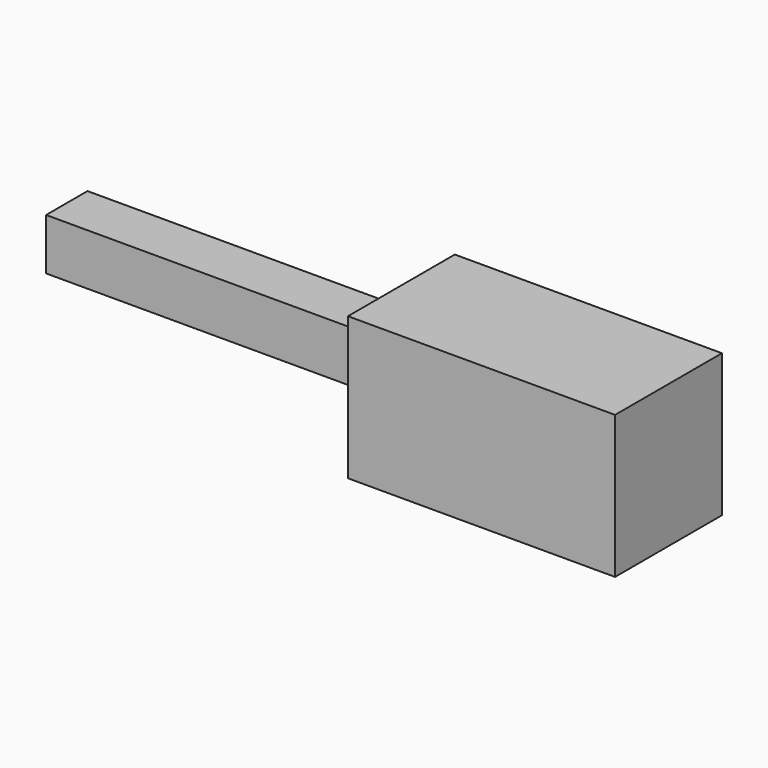
from build123d import *

# Parameters (mm, degrees)
F0_W     = 50.8
F0_H     = 27.1318203053
F1_DEPTH = 25.4
F2_DEPTH = 25.4
F4_W     = 9.8461210728
F4_H     = 9.7858998924
F5_DEPTH = 62.9539089


# Not quite as in the source:
# - an extrude ends at something that could not be found from the text; its depth is read off the source's solid


with BuildPart() as f1:
    # F0 (on Front) → F1 (new body)
    with BuildSketch(Plane.XZ):
        with Locations((-45.1160669327, 19.4199038669)):
            Rectangle(F0_W, F0_H)
    extrude(amount=F1_DEPTH)

    # F2 (add): a face of the model
    f2_faces = [f1.faces().sort_by_distance(p)[0] for p in [
        (-70.5160669327, -12.7, 19.4199038669),
    ]]
    extrude(f2_faces, amount=-F2_DEPTH)

    # F4 (on face) → F5 (join, through all)
    with BuildSketch(Plane(origin=(-70.5160669327, 0, 0), x_dir=(0, -1, 0), z_dir=(-1, 0, 0))):
        with Locations((13.5363917798, 21.7452598736)):
            Rectangle(F4_W, F4_H)
    extrude(amount=F5_DEPTH)


solid = f1.part
